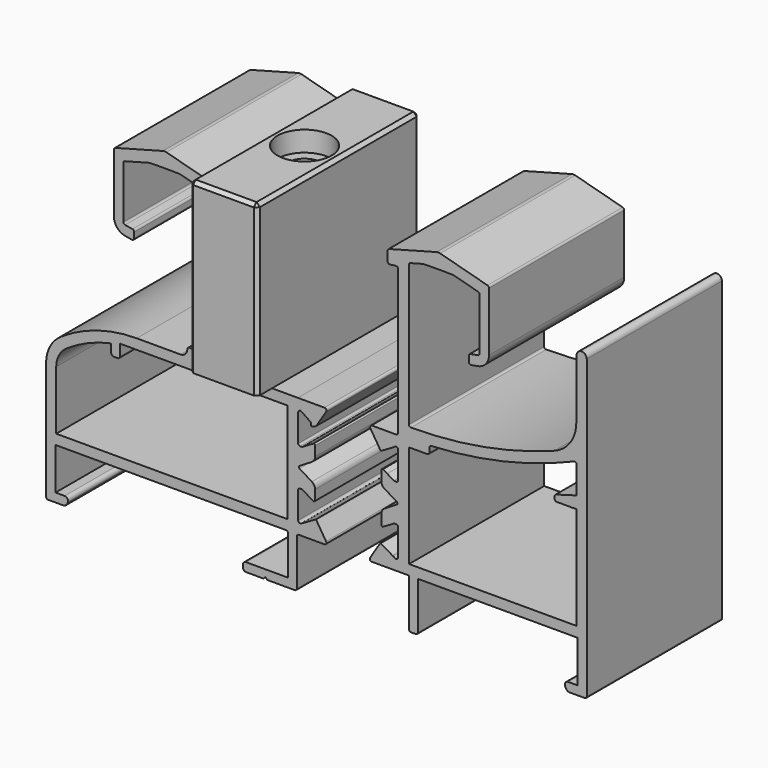
from build123d import *

# Parameters (mm, degrees)
F0_W           = 10
F0_H           = 25
F1_DEPTH       = 30
F3_D           = 5
F3_DEPTH       = 22
F3_CBORE_D     = 8
F3_CBORE_DEPTH = 3
F3_TIP         = 1.5021515476
F4_DEPTH       = 25
F5_SIZE        = 0.5


# Not quite as in the source:
# - ends of sketch curves that miss each other by under 0.0002 mm in the source are joined


with BuildPart() as f1:
    # F0 (on Front) → F1 (new body)
    with BuildSketch(Plane.XZ):
        with Locations((-9.7568192333, 13.8142455369)):
            Rectangle(F0_W, F0_H)
    extrude(amount=F1_DEPTH)

    # F3
    with Locations(Plane.XY.offset(26.3142455369)):
        with Locations((-9.7568192333, -15)):
            CounterBoreHole(F3_D / 2, F3_CBORE_D / 2, F3_CBORE_DEPTH, depth=F3_DEPTH)
            with Locations((0, 0, -(F3_DEPTH + F3_TIP / 2))):  # 118° drill point
                Cone(0, F3_D / 2, F3_TIP, mode=Mode.SUBTRACT)

    # F5
    f5_edges = [f1.edges().sort_by_distance(p)[0] for p in [
        (-9.756819, -30, 26.314246),
        (-14.756819, -30, 13.814246),
        (-4.756819, -30, 13.814246),
        (-14.756819, -15, 26.314246),
        (-4.756819, -15, 26.314246),
        (-9.756819, 0, 26.314246),
        (-4.756819, 0, 13.814246),
        (-14.756819, 0, 13.814246),
    ]]
    chamfer(f5_edges, length=F5_SIZE)


with BuildPart() as f4:
    # F0 (on Front) → F4 (new body)
    with BuildSketch(Plane.XZ):
        with BuildLine():
            Line((-0.1939404092, -3.0787518674), (-1.2332873744, -2.4786841638))
            Line((-1.2332873744, -2.4786841638), (-0.906405, -2.701009))
            ThreePointArc((-0.906405, -2.701009), (-0.8387871919, -2.7794041179), (-0.8194255026, -2.8811049629))
            Line((-0.8194255026, -2.8811049629), (-0.832174, -3.05384))
            ThreePointArc((-0.832174, -3.05384), (-0.7451945613, -3.2339357206), (-0.5457370974, -3.2486567983))
            Line((-0.5457370974, -3.2486567983), (-0.1939404092, -3.0787518674))
        make_face()
        with BuildLine():
            Line((-2.698738, -12.435705), (-2.698738, -12.189499))
            ThreePointArc((-2.698738, -12.189499), (-2.6196568309, -11.9985801691), (-2.428738, -11.919499))
            Line((-2.428738, -11.919499), (-2.154956, -11.919499))
            ThreePointArc((-2.154956, -11.919499), (-2.1008358406, -11.9269606705), (-2.0507539491, -11.9487889166))
            Line((-2.0507539491, -11.9487889166), (-1.3911990793, -12.3513827296))
            Line((-1.3911990793, -12.3513827296), (-0.4072709459, -12.9194543316))
            ThreePointArc((-0.4072709459, -12.9194543316), (-0.2600806177, -12.8611433227), (-0.198739, -12.71519))
            Line((-0.198739, -12.71519), (-0.198738, -11.297285))
            ThreePointArc((-0.198738, -11.297285), (-0.3266688854, -10.807902267), (-0.6777289186, -10.4437338667))
            Line((-0.6777289186, -10.4437338667), (-2.50294, -9.32962))
            ThreePointArc((-2.50294, -9.32962), (-2.5731518902, -9.2567864267), (-2.598738, -9.15891))
            ThreePointArc((-2.598738, -9.15891), (-2.5731518902, -9.0610335733), (-2.5029400509, -8.9881999166))
            Line((-2.5029400509, -8.9881999166), (-0.677729, -7.874086))
            ThreePointArc((-0.677729, -7.874086), (-0.3266688854, -7.509917733), (-0.198738, -7.020535))
            Line((-0.198738, -7.020535), (-0.198738, -5.60263))
            ThreePointArc((-0.198738, -5.60263), (-0.2675198615, -5.4497439195), (-0.4275519061, -5.3997968951))
            Line((-0.4275519061, -5.3997968951), (-1.0802291409, -5.7766205571))
            Line((-1.0802291409, -5.7766205571), (-2.050754, -6.369031))
            ThreePointArc((-2.050754, -6.369031), (-2.1008358406, -6.3908593295), (-2.154956, -6.398321))
            Line((-2.154956, -6.398321), (-2.428738, -6.398321))
            ThreePointArc((-2.428738, -6.398321), (-2.6196568309, -6.3192398309), (-2.698738, -6.128321))
            Line((-2.698738, -6.128321), (-2.698738, -5.871837))
            Line((-2.698738, -5.871837), (-2.698738, -2.471837))
            Line((-2.698738, -2.471837), (-2.698738, -2.04883))
            ThreePointArc((-2.698738, -2.04883), (-2.6932284845, -2.0301461988), (-2.689562667, -2.0110150471))
            ThreePointArc((-2.689562667, -2.0110150471), (-2.5138811939, -1.7786992249), (-2.2238068542, -1.8049947857))
            Line((-2.2238068542, -1.8049947857), (-1.2332873744, -2.4786841638))
            Line((-1.2332873744, -2.4786841638), (-0.1939404092, -3.0787518674))
            Line((-0.1939404092, -3.0787518674), (-0.094366, -3.030661))
            ThreePointArc((-0.094366, -3.030661), (-0.0480939665, -2.9997097688), (-0.0121459252, -2.9572030471))
            Line((-0.0121459252, -2.9572030471), (1.435188, -0.66075))
            ThreePointArc((1.435188, -0.66075), (1.4441046934, -0.3559466522), (1.181594, -0.20079307))
            Line((1.181594, -0.20079307), (-2.749431, -0.198321))
            Line((-2.749431, -0.198321), (-16.007338, -0.198321))
            ThreePointArc((-16.007338, -0.198321), (-16.3608913906, -0.0518743906), (-16.507338, 0.301679))
            Line((-16.507338, 0.301679), (-16.507338, 21.413958))
            ThreePointArc((-16.507338, 21.413958), (-16.4063795658, 21.6384183642), (-16.171454966, 21.7118042823))
            Line((-16.171454966, 21.7118042823), (-15.257338, 21.601679))
            ThreePointArc((-15.257338, 21.601679), (-15.0452059656, 21.6895469656), (-14.957338, 21.901679))
            Line((-14.957338, 21.901679), (-14.957338, 23.29378))
            ThreePointArc((-14.957338, 23.29378), (-15.0193319335, 23.4764083448), (-15.1796920822, 23.5835576932))
            Line((-15.1796920822, 23.5835576932), (-22.198519, 25.464247))
            ThreePointArc((-22.198519, 25.464247), (-22.457338, 25.498321), (-22.7161569596, 25.4642468492))
            Line((-22.7161569596, 25.4642468492), (-29.734983, 23.583558))
            ThreePointArc((-29.734983, 23.583558), (-29.8953437724, 23.476408728), (-29.957338, 23.29378))
            Line((-29.957338, 23.29378), (-29.957338, 14.560928))
            ThreePointArc((-29.957338, 14.560928), (-29.4894267462, 13.2753526137), (-28.3046339262, 12.5913124183))
            Line((-28.3046339262, 12.5913124183), (-27.310551, 12.416028))
            ThreePointArc((-27.310551, 12.416028), (-27.0656198785, 12.4816575316), (-26.958456, 12.711471))
            Line((-26.958456, 12.711471), (-26.958456, 13.523812))
            ThreePointArc((-26.958456, 13.523812), (-27.0286427924, 13.7166484322), (-27.2063619306, 13.8192543936))
            Line((-27.2063619306, 13.8192543936), (-28.309432, 14.013755))
            ThreePointArc((-28.309432, 14.013755), (-28.4871511518, 14.1163615013), (-28.557338, 14.309198))
            Line((-28.557338, 14.309198), (-28.557338, 22.012467))
            ThreePointArc((-28.557338, 22.012467), (-28.4953437724, 22.195095728), (-28.3349829848, 22.3022449432))
            Line((-28.3349829848, 22.3022449432), (-24.761014, 23.259887))
            ThreePointArc((-24.761014, 23.259887), (-24.7022805215, 23.2719037679), (-24.6425309914, 23.2768046085))
            ThreePointArc((-24.6425309914, 23.2768046085), (-22.457338, 23.300683), (-20.2721450042, 23.276804807))
            ThreePointArc((-20.2721450042, 23.276804807), (-20.2123950004, 23.2719036997), (-20.1536610537, 23.2598867996))
            Line((-20.1536610537, 23.2598867996), (-18.329692, 22.771156))
            ThreePointArc((-18.329692, 22.771156), (-18.1693318548, 22.6640072422), (-18.107338, 22.481379))
            Line((-18.107338, 22.481379), (-18.107338, 1.401679))
            ThreePointArc((-18.107338, 1.401679), (-18.1952059656, 1.1895469656), (-18.407338, 1.101679))
            Line((-18.407338, 1.101679), (-18.805937, 1.101679))
            ThreePointArc((-18.805937, 1.101679), (-19.0180690344, 1.0138110344), (-19.105937, 0.801679))
            ThreePointArc((-19.105937, 0.801679), (-19.3988302188, 0.0945722188), (-20.105937, -0.198321))
            Line((-20.105937, -0.198321), (-26.582989, -0.198321))
            ThreePointArc((-26.582989, -0.198321), (-32.4538230596, -1.0793956263), (-37.8073928267, -3.6449902556))
            ThreePointArc((-37.8073928267, -3.6449902556), (-39.4188999928, -5.4413709036), (-40.001292, -7.783327))
            Line((-40.001292, -7.783327), (-40.001278, -25.198321))
            ThreePointArc((-40.001278, -25.198321), (-39.9134100344, -25.4104530344), (-39.701278, -25.498321))
            Line((-39.701278, -25.498321), (-37.424497, -25.498321))
            ThreePointArc((-37.424497, -25.498321), (-37.174502259, -25.4313374702), (-36.9914897369, -25.2483331519))
            Line((-36.9914897369, -25.2483331519), (-36.818271, -24.94833))
            ThreePointArc((-36.818271, -24.94833), (-36.8182596124, -24.4483261161), (-37.251272, -24.198318))
            Line((-37.251272, -24.198318), (-38.601285, -24.198303))
            Line((-38.601285, -24.198303), (-38.601285, -17.998321))
            Line((-38.601285, -17.998321), (-4.498738, -17.998321))
            ThreePointArc((-4.498738, -17.998321), (-4.2866059656, -18.0861889656), (-4.198738, -18.298321))
            Line((-4.198738, -18.298321), (-4.198738, -24.098318))
            Line((-4.198738, -24.098318), (-10.398738, -24.098318))
            ThreePointArc((-10.398738, -24.098318), (-10.7522913906, -24.2447646094), (-10.898738, -24.598318))
            Line((-10.898738, -24.598318), (-10.898738, -24.898321))
            ThreePointArc((-10.898738, -24.898321), (-10.7522913906, -25.2518743906), (-10.398738, -25.398321))
            Line((-10.398738, -25.398321), (-7.848738, -25.398321))
            Line((-7.848738, -25.398321), (-7.548738, -25.098321))
            Line((-7.548738, -25.098321), (-7.248738, -25.398321))
            Line((-7.248738, -25.398321), (-3.198738, -25.398321))
            ThreePointArc((-3.198738, -25.398321), (-2.9866059656, -25.3104530344), (-2.898738, -25.098321))
            Line((-2.898738, -25.098321), (-2.898738, -18.298321))
            ThreePointArc((-2.898738, -18.298321), (-2.8108700344, -18.0861889656), (-2.598738, -17.998321))
            Line((-2.598738, -17.998321), (1.172522, -17.998321))
            ThreePointArc((1.172522, -17.998321), (1.4351385761, -17.8433469769), (1.4264301699, -17.5385378931))
            Line((1.4264301699, -17.5385378931), (-0.019336, -15.241098))
            ThreePointArc((-0.019336, -15.241098), (-0.051798309, -15.2017336236), (-0.0931641553, -15.1718636868))
            ThreePointArc((-0.0931641553, -15.1718636868), (-0.1156977491, -15.1839305506), (-0.1379692098, -15.1964746366))
            Line((-0.1379692098, -15.1964746366), (-1.845148, -16.182115))
            ThreePointArc((-1.845148, -16.182115), (-1.9188980977, -16.2152586354), (-1.9978068205, -16.2328936362))
            Line((-1.9978068205, -16.2328936362), (-2.230191, -16.390715))
            ThreePointArc((-2.230191, -16.390715), (-2.5391588236, -16.4076445108), (-2.698738, -16.142537))
            Line((-2.698738, -16.142537), (-2.698738, -15.835705))
            Line((-2.698738, -15.835705), (-2.698738, -12.435705))
        make_face()
        with BuildLine():
            Line((-30.398738, -2.09611), (-30.398738, -3.198321))
            ThreePointArc((-30.398738, -3.198321), (-30.2522913906, -3.5518743906), (-29.898738, -3.698321))
            Line((-29.898738, -3.698321), (-29.398738, -3.698321))
            ThreePointArc((-29.398738, -3.698321), (-29.1866059656, -3.6104530344), (-29.098738, -3.398321))
            Line((-29.098738, -3.398321), (-29.098738, -1.698321))
            Line((-29.098738, -1.698321), (-4.298738, -1.698321))
            Line((-4.298738, -1.698321), (-4.298738, -16.498321))
            Line((-4.298738, -16.498321), (-38.501285, -16.498321))
            Line((-38.501285, -16.498321), (-38.501292, -7.783326))
            ThreePointArc((-38.501292, -7.783326), (-38.0936177131, -6.1439567553), (-36.9655628403, -4.8864902355))
            ThreePointArc((-36.9655628403, -4.8864902355), (-33.8179492297, -3.1717138666), (-30.398738, -2.09611))
        make_face(mode=Mode.SUBTRACT)
    extrude(amount=F4_DEPTH)


with BuildPart() as f4b:
    # F0 (on Front) → F4, piece 2 (new body)
    with BuildSketch(Plane.XZ):
        with BuildLine():
            ThreePointArc((9.601262, -12.71519), (9.6626036762, -12.8611433799), (9.8097941095, -12.9194543282))
            Line((9.8097941095, -12.9194543282), (10.7937171592, -12.3513859941))
            Line((10.7937171592, -12.3513859941), (11.453277, -11.948789))
            ThreePointArc((11.453277, -11.948789), (11.5033588406, -11.9269606705), (11.557479, -11.919499))
            Line((11.557479, -11.919499), (11.831262, -11.919499))
            ThreePointArc((11.831262, -11.919499), (12.0221808309, -11.9985801691), (12.101262, -12.189499))
            Line((12.101262, -12.189499), (12.101262, -12.435705))
            Line((12.101262, -12.435705), (12.101262, -15.835705))
            Line((12.101262, -15.835705), (12.101262, -16.161459))
            ThreePointArc((12.101262, -16.161459), (11.9416828236, -16.4265665108), (11.6327153847, -16.4096364335))
            Line((11.6327153847, -16.4096364335), (11.3633839308, -16.2267235691))
            ThreePointArc((11.3633839308, -16.2267235691), (11.3037886621, -16.2089309169), (11.2476719301, -16.1821151211))
            Line((11.2476719301, -16.1821151211), (9.540492, -15.196475))
            ThreePointArc((9.540492, -15.196475), (9.5114299913, -15.1802288941), (9.481928255, -15.1647956753))
            Line((9.481928255, -15.1647956753), (9.476167, -15.167583))
            ThreePointArc((9.476167, -15.167583), (9.4299166933, -15.1985666686), (9.3939978867, -15.2410979287))
            Line((9.3939978867, -15.2410979287), (7.948231, -17.538538))
            ThreePointArc((7.948231, -17.538538), (7.9395235526, -17.84334721), (8.20214, -17.998321))
            Line((8.20214, -17.998321), (12.534078, -17.998321))
            Line((12.534078, -17.998321), (13.701292, -17.998321))
            Line((13.701292, -17.998321), (13.701292, -24.998321))
            ThreePointArc((13.701292, -24.998321), (13.7891599656, -25.2104530344), (14.001292, -25.298321))
            Line((14.001292, -25.298321), (14.701292, -25.298321))
            ThreePointArc((14.701292, -25.298321), (14.9134240344, -25.2104530344), (15.001292, -24.998321))
            Line((15.001292, -24.998321), (15.001292, -17.998321))
            Line((15.001292, -17.998321), (38.601299, -17.998321))
            Line((38.601299, -17.998321), (38.601299, -24.198303))
            Line((38.601299, -24.198303), (37.251286, -24.198318))
            ThreePointArc((37.251286, -24.198318), (36.8182736124, -24.4483261161), (36.8182851699, -24.9483299019))
            Line((36.8182851699, -24.9483299019), (36.991504, -25.248333))
            ThreePointArc((36.991504, -25.248333), (37.174516259, -25.4313374702), (37.424511, -25.498321))
            Line((37.424511, -25.498321), (39.701292, -25.498321))
            ThreePointArc((39.701292, -25.498321), (39.9134240344, -25.4104530344), (40.001292, -25.198321))
            Line((40.001292, -25.198321), (40.001256, 18.752611))
            ThreePointArc((40.001256, 18.752611), (39.2512585, 19.502607), (38.501262, 18.75261))
            Line((38.501262, 18.75261), (38.448763, 9.902302))
            ThreePointArc((38.448763, 9.902302), (37.5539777797, 7.0775023608), (35.2174500545, 5.2552038559))
            ThreePointArc((35.2174500545, 5.2552038559), (24.7808442556, 2.3538398503), (13.992654, 1.3762900215))
            ThreePointArc((13.992654, 1.3762900215), (13.7805271372, 1.4641607941), (13.692662, 1.67629))
            Line((13.692662, 1.67629), (13.692662, 22.481379))
            ThreePointArc((13.692662, 22.481379), (13.7546561488, 22.6640076253), (13.9150167652, 22.7711568762))
            Line((13.9150167652, 22.7711568762), (15.738986, 23.259887))
            ThreePointArc((15.738986, 23.259887), (15.7977194785, 23.2719037679), (15.8574690086, 23.2768046085))
            ThreePointArc((15.8574690086, 23.2768046085), (18.042662, 23.300683), (20.2278549958, 23.276804807))
            ThreePointArc((20.2278549958, 23.276804807), (20.2876049996, 23.2719036997), (20.3463389463, 23.2598867996))
            Line((20.3463389463, 23.2598867996), (23.920308, 22.302245))
            ThreePointArc((23.920308, 22.302245), (24.0806680665, 22.1950953448), (24.142662, 22.012467))
            Line((24.142662, 22.012467), (24.142662, 14.309198))
            ThreePointArc((24.142662, 14.309198), (24.0724754684, 14.1163618785), (23.8947568682, 14.0137557473))
            Line((23.8947568682, 14.0137557473), (22.791686, 13.819254))
            ThreePointArc((22.791686, 13.819254), (22.6139674758, 13.716648055), (22.543781, 13.523812))
            Line((22.543781, 13.523812), (22.543781, 12.711471))
            ThreePointArc((22.543781, 12.711471), (22.6509445013, 12.4816578482), (22.8958748984, 12.4160285763))
            Line((22.8958748984, 12.4160285763), (23.889959, 12.591312))
            ThreePointArc((23.889959, 12.591312), (25.0747510627, 13.2753529909), (25.542662, 14.560928))
            Line((25.542662, 14.560928), (25.542662, 23.29378))
            ThreePointArc((25.542662, 23.29378), (25.4806680665, 23.4764083448), (25.3203079178, 23.5835576932))
            Line((25.3203079178, 23.5835576932), (18.301481, 25.464247))
            ThreePointArc((18.301481, 25.464247), (18.042662, 25.498321), (17.7838430404, 25.4642468492))
            Line((17.7838430404, 25.4642468492), (10.765017, 23.583558))
            ThreePointArc((10.765017, 23.583558), (10.6046562276, 23.476408728), (10.542662, 23.29378))
            Line((10.542662, 23.29378), (10.542662, 21.901679))
            ThreePointArc((10.542662, 21.901679), (10.6305299656, 21.6895469656), (10.842662, 21.601679))
            Line((10.842662, 21.601679), (11.75678, 21.711804))
            ThreePointArc((11.75678, 21.711804), (11.9917039372, 21.6384180349), (12.092662, 21.413958))
            Line((12.092662, 21.413958), (12.092662, 0.052573))
            ThreePointArc((12.092662, 0.052573), (12.0047940344, -0.1595590344), (11.792662, -0.247427))
            Line((11.792662, -0.247427), (8.250563, -0.247427))
            ThreePointArc((8.250563, -0.247427), (7.9879464239, -0.4024010231), (7.9966548301, -0.7072101069))
            Line((7.9966548301, -0.7072101069), (9.442421, -3.00465))
            ThreePointArc((9.442421, -3.00465), (9.4783398665, -3.0471814863), (9.5245906948, -3.0781646308))
            Line((9.5245906948, -3.0781646308), (9.5642490125, -3.0973508801))
            Line((9.5642490125, -3.0973508801), (11.247672, -2.125426))
            ThreePointArc((11.247672, -2.125426), (11.2633381751, -2.1168425761), (11.2793716222, -2.1089665234))
            Line((11.2793716222, -2.1089665234), (11.632715, -1.868997))
            ThreePointArc((11.632715, -1.868997), (11.9416825754, -1.8520663577), (12.101262, -2.117174))
            Line((12.101262, -2.117174), (12.101262, -2.471837))
            Line((12.101262, -2.471837), (12.101262, -5.871837))
            Line((12.101262, -5.871837), (12.101262, -6.128321))
            ThreePointArc((12.101262, -6.128321), (12.0221808309, -6.3192398309), (11.831262, -6.398321))
            Line((11.831262, -6.398321), (11.557479, -6.398321))
            ThreePointArc((11.557479, -6.398321), (11.5033588406, -6.3908593295), (11.4532769491, -6.3690310834))
            Line((11.4532769491, -6.3690310834), (10.4827541288, -5.7766213861))
            Line((10.4827541288, -5.7766213861), (9.8300751206, -5.399796921))
            ThreePointArc((9.8300751206, -5.399796921), (9.6700429424, -5.4497438479), (9.601262, -5.60263))
            Line((9.601262, -5.60263), (9.601262, -7.020535))
            ThreePointArc((9.601262, -7.020535), (9.7291926765, -7.5099173608), (10.0802521901, -7.8740856886))
            Line((10.0802521901, -7.8740856886), (11.905464, -8.9882))
            ThreePointArc((11.905464, -8.9882), (11.9756758902, -9.0610335733), (12.001262, -9.15891))
            ThreePointArc((12.001262, -9.15891), (11.9756758902, -9.2567864267), (11.9054640509, -9.3296200834))
            Line((11.9054640509, -9.3296200834), (10.080252, -10.443734))
            ThreePointArc((10.080252, -10.443734), (9.7291926765, -10.8079026392), (9.601262, -11.297285))
            Line((9.601262, -11.297285), (9.601262, -12.71519))
        make_face()
        with BuildLine():
            Line((38.501262, -16.497393), (13.701262, -16.497393))
            Line((13.701262, -16.497393), (13.701262, -1.297393))
            Line((13.701262, -1.297393), (16.401262, -1.297393))
            ThreePointArc((16.401262, -1.297393), (16.6133940344, -1.2095250344), (16.701262, -0.997393))
            Line((16.701262, -0.997393), (16.701262, -0.350511))
            ThreePointArc((16.701262, -0.350511), (16.7840304303, -0.1436041487), (16.9866649675, -0.0508663327))
            ThreePointArc((16.9866649675, -0.0508663327), (27.7498829967, 1.434377589), (38.0837561049, 4.7905477535))
            ThreePointArc((38.0837561049, 4.7905477535), (38.366715822, 4.7647725852), (38.501266, 4.514519))
            Line((38.501266, 4.514519), (38.501262, 0.502607))
            Line((38.501262, 0.502607), (35.471557, -0.366959))
            ThreePointArc((35.471557, -0.366959), (35.3134338404, -0.4745587226), (35.252466, -0.655842))
            Line((35.252466, -0.655842), (35.252466, -0.997393))
            ThreePointArc((35.252466, -0.997393), (35.3403339656, -1.2095250344), (35.552466, -1.297393))
            Line((35.552466, -1.297393), (38.501262, -1.297393))
            Line((38.501262, -1.297393), (38.501262, -16.497393))
        make_face(mode=Mode.SUBTRACT)
    extrude(amount=F4_DEPTH)


solid = Compound([f1.part, f4.part, f4b.part])
